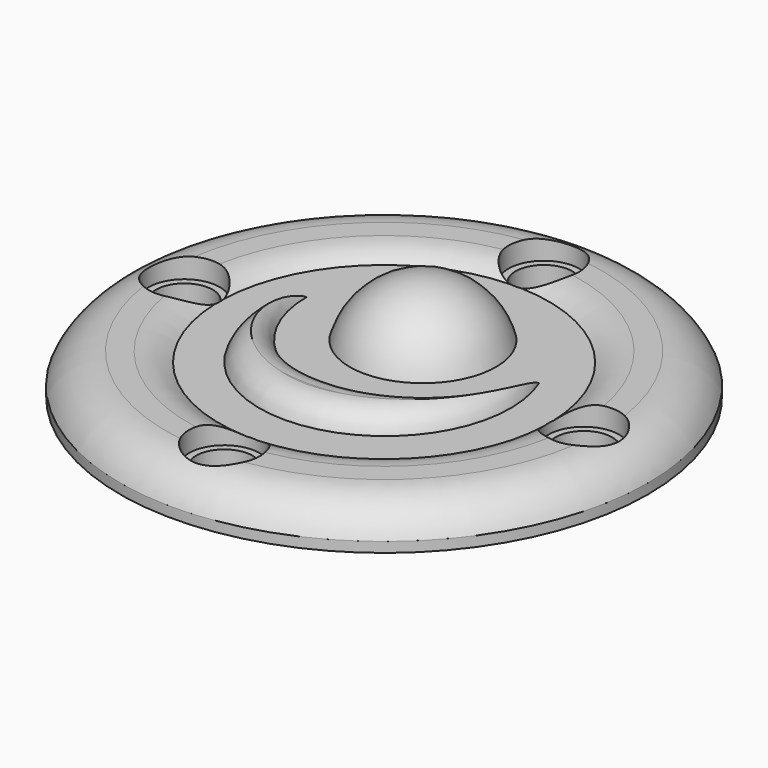
from build123d import *

# Parameters (mm, degrees)
F0_R        = 26.1
F1_DEPTH    = 3
F2_R        = 16.3023270164
F3_DEPTH    = 1
F5_R        = 2.8
F6_DEPTH    = 3.0010001
F8_DEPTH    = 2
F9_T2_ANGLE = 247.8747937478
F9_T4_ANGLE = 287.2551612694
F11_R       = 3.5
F12_DEPTH   = 2
F14_ANGLE   = 180
F16_R       = 26.1
F16_R_2     = 2.8
F17_DEPTH   = 1


# Not quite as in the source:
# - a fillet or chamfer that OpenCascade refuses, or shapes differently, is made with other operations: its cross-section is extruded or revolved along the edge and cut away or added


with BuildPart() as f1:
    # F0 (on Top) → F1 (new body)
    with BuildSketch(Plane.XY):
        Circle(F0_R)
    extrude(amount=F1_DEPTH)

    # F2 (on face) → F3 (cut)
    with BuildSketch(Plane.XY.offset(3)):
        Circle(F2_R)
    extrude(amount=-F3_DEPTH, mode=Mode.SUBTRACT)

    # F4: fillet of radius 5 on 2 edges, made by hand

    # F4_s1 → F4_t2 (revolve, cut)
    with BuildSketch(Plane.XZ):
        with BuildLine():
            ThreePointArc((26.1, 0), (24.2560370926, 2.1833001327), (21.517424305, 3))
            Line((21.517424305, 3), (26.1, 3))
            Line((26.1, 3), (26.1, 0))
        make_face()
    revolve(axis=Axis((0, 0, 3), (0, 0, 1)), mode=Mode.SUBTRACT)

    # F4_s3 → F4_t4 (revolve, cut)
    with BuildSketch(Plane.XZ):
        with BuildLine():
            ThreePointArc((19.3023270164, 3), (17.7211881863, 2.7434164903), (16.3023270164, 2))
            Line((16.3023270164, 2), (16.3023270164, 3))
            Line((16.3023270164, 3), (19.3023270164, 3))
        make_face()
    revolve(axis=Axis((0, 0, 3), (0, 0, 1)), mode=Mode.SUBTRACT)

    # F5 (on Top) → F6 (cut, through all)
    with BuildSketch(Plane.XY):
        with Locations((0, 19.75)):
            Circle(F5_R)
        with Locations((-19.75, 0)):
            Circle(F5_R)
        with Locations((0, -19.75)):
            Circle(F5_R)
        with Locations((19.75, 0)):
            Circle(F5_R)
    extrude(amount=F6_DEPTH, mode=Mode.SUBTRACT)

    # F7 (on face) → F8 (join)
    with BuildSketch(Plane.XY.offset(2)):
        with BuildLine():
            ThreePointArc((11.5, 4.8023270164), (0, -6.6976729836), (-11.5, 4.8023270164))
            ThreePointArc((-11.5, 4.8023270164), (0, -12.3023270164), (11.5, 4.8023270164))
        make_face()
    extrude(amount=F8_DEPTH)

    # F9: fillet of radius 2.85 on 2 edges, made by hand

    # F9_s1 → F9_t2 (revolve, cut)
    with BuildSketch(Plane(origin=(-2.2243490984, 3.3055181298, 0), x_dir=(0, 0, 1), z_dir=(-0.558286738, 0.8296480689, 0))):
        with BuildLine():
            ThreePointArc((2, 14.1810754847), (3.4461925006, 15.2131752848), (4, 16.9013695864))
            Line((4, 16.9013695864), (4, 14.1810754847))
            Line((4, 14.1810754847), (2, 14.1810754847))
        make_face()
    revolve(axis=Axis((0, 4.8023270164, 4), (0, 0, -1)), revolution_arc=F9_T2_ANGLE, mode=Mode.SUBTRACT)

    # F9_s3 → F9_t4 (revolve, cut)
    with BuildSketch(Plane(origin=(0.0553451509, 0.0407628561, 0), x_dir=(0, 0, 1), z_dir=(0.8051793599, 0.5930313638, 0))):
        with BuildLine():
            ThreePointArc((2, -12.5115597549), (3.4461925006, -11.4794599548), (4, -9.7912656532))
            Line((4, -9.7912656532), (4, -12.5115597549))
            Line((4, -12.5115597549), (2, -12.5115597549))
        make_face()
    revolve(axis=Axis((0, 0.1159068972, 4), (0, 0, 1)), revolution_arc=F9_T4_ANGLE, mode=Mode.SUBTRACT)

    # F11 (on offset) → F12 (cut)
    with BuildSketch(Plane.XY.offset(3)):
        with Locations((0, 19.75)):
            Circle(F11_R)
        with Locations((19.75, 0)):
            Circle(F11_R)
        with Locations((0, -19.75)):
            Circle(F11_R)
        with Locations((-19.75, 0)):
            Circle(F11_R)
    extrude(amount=-F12_DEPTH, mode=Mode.SUBTRACT)

    # F13 (on Top) → F14 (revolve)
    with BuildSketch(Plane.XY):
        with BuildLine():
            Line((0, 12.3023270164), (0, -2.6976729836))
            ThreePointArc((0, -2.6976729836), (7.5, 4.8023270164), (0, 12.3023270164))
        make_face()
    revolve(axis=Axis((0, 4.8023270164, 0), (0, -1, 0)), revolution_arc=F14_ANGLE)


with BuildPart() as f1_1:
    # F15: moved
    add(f1.part.moved(Location((0, 0, 1))))

    # F16 (on face) → F17 (join)
    with BuildSketch(Plane(origin=(0, 0, 1), x_dir=(1, 0, 0), z_dir=(0, 0, -1))):
        Circle(F16_R)
        with Locations((0, -19.75)):
            Circle(F16_R_2, mode=Mode.SUBTRACT)
        with Locations((-19.75, 0)):
            Circle(F16_R_2, mode=Mode.SUBTRACT)
        with Locations((19.75, 0)):
            Circle(F16_R_2, mode=Mode.SUBTRACT)
        with Locations((0, 19.75)):
            Circle(F16_R_2, mode=Mode.SUBTRACT)
    extrude(amount=F17_DEPTH)


solid = f1_1.part
